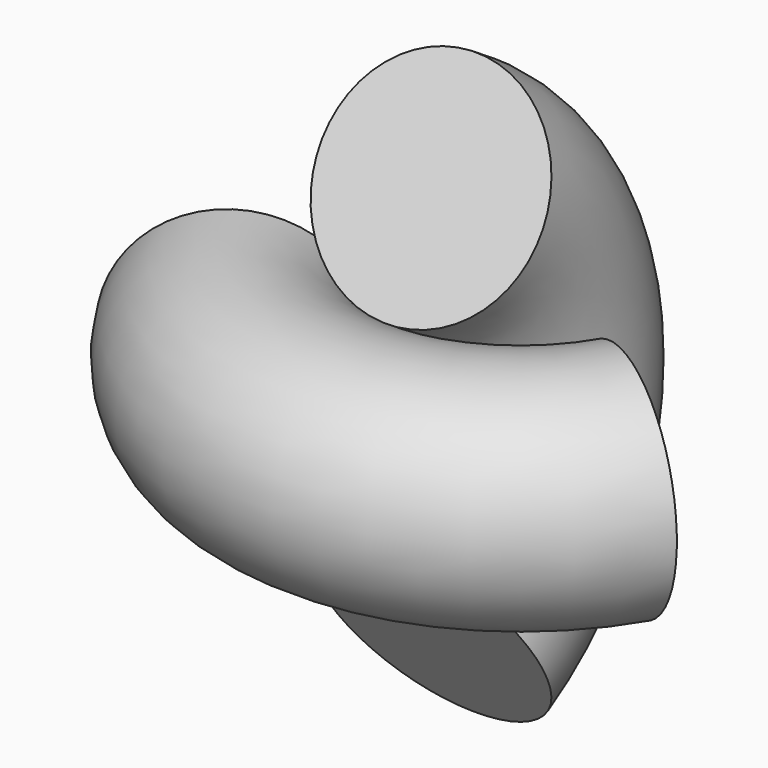
from build123d import *

# Parameters (mm, degrees)
F0_R          = 9.525
F1_ANGLE_BACK = 60
F1_ANGLE      = 120
F2_R          = 9.525
F3_ANGLE_BACK = 60
F3_ANGLE      = 120


with BuildPart() as f1:
    # F0 (on Right) → F1 (revolve)
    with BuildSketch(Plane.YZ, mode=Mode.PRIVATE) as f1_sk:
        with Locations((-19.05, 0)):
            Circle(F0_R)
    revolve(f1_sk.sketch.rotate(Axis((0, 0, 8.618671447), (0, 0, -1)), -F1_ANGLE_BACK), axis=Axis((0, 0, 8.618671447), (0, 0, -1)), revolution_arc=F1_ANGLE)


with BuildPart() as f3:
    # F2 (on Top) → F3 (revolve)
    with BuildSketch(Plane.XY, mode=Mode.PRIVATE) as f3_sk:
        Circle(F2_R)
    revolve(f3_sk.sketch.rotate(Axis((9.3368953094, -19.05, 0), (1, 0, 0)), -F3_ANGLE_BACK), axis=Axis((9.3368953094, -19.05, 0), (1, 0, 0)), revolution_arc=F3_ANGLE)


solid = Compound([f1.part, f3.part])
